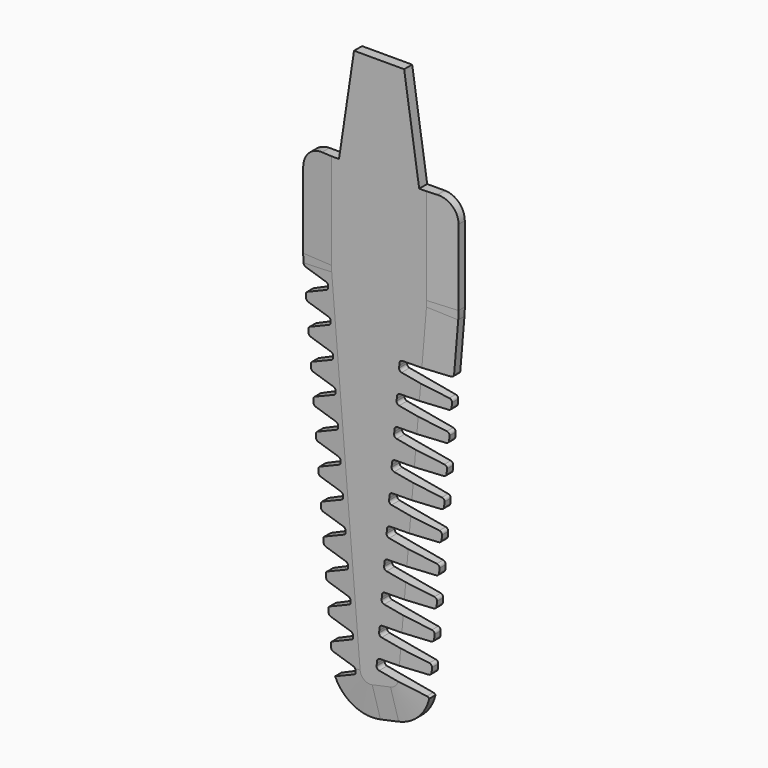
from build123d import *

# Parameters (mm, degrees)
F1_DEPTH    = 0.635
F2_T1_DEPTH = 3.9112557533
F3_R        = 2.54
F4_R        = 5.08
F11_DEPTH   = 12.7
F13_DEPTH   = 12.7
F15_DEPTH   = 12.7
F17_DEPTH   = 0.635
F20_DEPTH   = 12.7


# Not quite as in the source:
# - a fillet or chamfer that OpenCascade refuses, or shapes differently, is made with other operations: its cross-section is extruded or revolved along the edge and cut away or added
# - two fillets or chamfers of one size are made in one step


with BuildPart() as f1:
    # F0 (on Front) → F1 (new body, symmetric)
    with BuildSketch(Plane.XZ):
        Polygon((-9.8425, -12.7), (-5.715, -62.23), (5.9259355188, -59.6987737741), (9.8425, -12.7), (9.8425, 0), (3.175, 0), (0, 0), (-3.175, 0), (-9.8425, 0), align=None)
    extrude(amount=F1_DEPTH, both=True)

    # F2: fillet of radius 12.7 on 2 edges, made by hand

    # F2_s2 → F2_t1 (cut)
    with BuildSketch(Plane.XZ.offset(-1.9556278767)):
        with BuildLine():
            ThreePointArc((-9.7986311297, -13.2264264435), (-9.8315280429, -12.6995436261), (-9.8425, -12.1717488493))
            Line((-9.8425, -12.1717488493), (-9.8425, -12.7))
            Line((-9.8425, -12.7), (-9.7986311297, -13.2264264435))
        make_face()
        with BuildLine():
            ThreePointArc((9.8425, -12.1717488493), (9.8315280429, -12.6995436261), (9.7986311297, -13.2264264435))
            Line((9.7986311297, -13.2264264435), (9.8425, -12.7))
            Line((9.8425, -12.7), (9.8425, -12.1717488493))
        make_face()
    extrude(amount=F2_T1_DEPTH, mode=Mode.SUBTRACT)

    # F3
    f3_edges = [f1.edges().sort_by_distance(p)[0] for p in [
        (9.8425, 0, 0),
        (-9.8425, 0, 0),
    ]]
    fillet(f3_edges, radius=F3_R)

    # F4
    f4_edges = [f1.edges().sort_by_distance(p)[0] for p in [
        (-5.715, 0, -62.23),
        (5.925936, 0, -59.698774),
    ]]
    fillet(f4_edges, radius=F4_R)


with BuildPart() as f8:
    # F8: sweep along a path in F7
    with BuildLine(Plane.XZ) as f8_path:
        Line((9.8425, 0), (9.8425, -12.1717488493))
        ThreePointArc((9.8425, -12.1717488493), (9.8315280429, -12.6995436261), (9.7986311297, -13.2264264435))
        Line((9.7986311297, -13.2264264435), (6.2379260636, -55.9548872367))
        ThreePointArc((6.2379260636, -55.9548872367), (4.9949337053, -58.8823630896), (2.2548556559, -60.4970200672))
        Line((2.2548556559, -60.4970200672), (-0.0542502185, -60.9991162551))
        ThreePointArc((-0.0542502185, -60.9991162551), (-4.1542208032, -60.1195272618), (-6.1960847146, -56.4569834247))
        Line((-6.1960847146, -56.4569834247), (-9.7986311297, -13.2264264435))
        ThreePointArc((-9.7986311297, -13.2264264435), (-9.8315280429, -12.6995436261), (-9.8425, -12.1717488493))
        Line((-9.8425, -12.1717488493), (-9.8425, 1.6673188657))
    # F6 (on Top) → F8 (sweep)
    with BuildSketch(Plane.XY):
        Polygon((9.8425, -0.635), (9.8425, -0.34925), (6.0325, -0.635), align=None)
    sweep(path=f8_path.line)


with BuildPart() as f1_1:
    add(f1.part)

    # F9: cut F8
    add(f8.part, mode=Mode.SUBTRACT)

    # F10 (on Front) → F11 (cut, symmetric)
    with BuildSketch(Plane.XZ):
        Polygon((5.8208333333, -60.96), (-5.715, -62.23), (5.715, -62.23), align=None)
    extrude(amount=F11_DEPTH, both=True, mode=Mode.SUBTRACT)

    # F12 (on Front) → F13 (cut, symmetric)
    with BuildSketch(Plane.XZ):
        with BuildLine():
            ThreePointArc((5.8493657763, -56.4687369075), (6.0838454994, -56.6117604145), (6.1612256866, -56.8752917613))
            Line((6.1612256866, -56.8752917613), (6.4296508148, -53.6541902219))
            ThreePointArc((6.4296508148, -53.6541902219), (6.3097189591, -53.9012788985), (6.0548005827, -54.0035192306))
            Line((6.0548005827, -54.0035192306), (0.1109684718, -54.0789339927))
            ThreePointArc((0.1109684718, -54.0789339927), (-0.1439499045, -54.1811743248), (-0.2638817603, -54.4282630014))
            Line((-0.2638817603, -54.4282630014), (-0.2878708353, -54.7161319011))
            Line((-0.2878708353, -54.7161319011), (-0.3118599102, -55.0040008009))
            ThreePointArc((-0.3118599102, -55.0040008009), (-0.2344797231, -55.2675321477), (0, -55.4105556547))
            Line((0, -55.4105556547), (5.8493657763, -56.4687369075))
        make_face()
    extrude(amount=F13_DEPTH, both=True, mode=Mode.SUBTRACT)

    # F14 (on Front) → F15 (cut, symmetric)
    with BuildSketch(Plane.XZ):
        with BuildLine():
            ThreePointArc((6.4296508148, -53.6541902219), (6.3097189591, -53.9012788985), (6.0548005827, -54.0035192306))
            Line((6.0548005827, -54.0035192306), (0.1109684718, -54.0789339927))
            ThreePointArc((0.1109684718, -54.0789339927), (-0.1439499045, -54.1811743248), (-0.2638817603, -54.4282630014))
            Line((-0.2638817603, -54.4282630014), (-0.2878708353, -54.7161319011))
            Line((-0.2878708353, -54.7161319011), (-0.3118599102, -55.0040008009))
            ThreePointArc((-0.3118599102, -55.0040008009), (-0.2344797231, -55.2675321477), (0, -55.4105556547))
            Line((0, -55.4105556547), (5.8493657763, -56.4687369075))
            ThreePointArc((5.8493657763, -56.4687369075), (6.0838454994, -56.6117604145), (6.1612256866, -56.8752917613))
            Line((6.1612256866, -56.8752917613), (6.4296508148, -53.6541902219))
        make_face()
        with BuildLine():
            Line((6.4776289648, -53.0784524224), (6.7460540931, -49.857350883))
            ThreePointArc((6.7460540931, -49.857350883), (6.6261222373, -50.1044395596), (6.371203861, -50.2066798917))
            Line((6.371203861, -50.2066798917), (0.4273717501, -50.2820946538))
            ThreePointArc((0.4273717501, -50.2820946538), (0.1724533737, -50.3843349859), (0.052521518, -50.6314236625))
            Line((0.052521518, -50.6314236625), (0.028532443, -50.9192925622))
            Line((0.028532443, -50.9192925622), (0.004543368, -51.207161462))
            ThreePointArc((0.004543368, -51.207161462), (0.0819235551, -51.4706928088), (0.3164032782, -51.6137163158))
            Line((0.3164032782, -51.6137163158), (6.1657690546, -52.6718975686))
            ThreePointArc((6.1657690546, -52.6718975686), (6.4002487777, -52.8149210756), (6.4776289648, -53.0784524224))
        make_face()
        with BuildLine():
            Line((6.794032243, -49.2816130835), (7.0624573713, -46.0605115441))
            ThreePointArc((7.0624573713, -46.0605115441), (6.9425255156, -46.3076002207), (6.6876071392, -46.4098405527))
            Line((6.6876071392, -46.4098405527), (0.7437750283, -46.4852553149))
            ThreePointArc((0.7437750283, -46.4852553149), (0.4888566519, -46.587495647), (0.3689247962, -46.8345843236))
            Line((0.3689247962, -46.8345843236), (0.3449357212, -47.1224532233))
            Line((0.3449357212, -47.1224532233), (0.3209466463, -47.4103221231))
            ThreePointArc((0.3209466463, -47.4103221231), (0.3983268334, -47.6738534699), (0.6328065565, -47.8168769769))
            Line((0.6328065565, -47.8168769769), (6.4821723328, -48.8750582297))
            ThreePointArc((6.4821723328, -48.8750582297), (6.7166520559, -49.0180817367), (6.794032243, -49.2816130835))
        make_face()
        with BuildLine():
            Line((7.1104355213, -45.4847737446), (7.3788606496, -42.2636722052))
            ThreePointArc((7.3788606496, -42.2636722052), (7.2589287938, -42.5107608818), (7.0040104175, -42.6130012138))
            Line((7.0040104175, -42.6130012138), (1.0601783066, -42.688415976))
            ThreePointArc((1.0601783066, -42.688415976), (0.8052599302, -42.7906563081), (0.6853280745, -43.0377449846))
            Line((0.6853280745, -43.0377449846), (0.6613389995, -43.3256138844))
            Line((0.6613389995, -43.3256138844), (0.6373499245, -43.6134827841))
            ThreePointArc((0.6373499245, -43.6134827841), (0.7147301116, -43.877014131), (0.9492098347, -44.020037638))
            Line((0.9492098347, -44.020037638), (6.7985756111, -45.0782188908))
            ThreePointArc((6.7985756111, -45.0782188908), (7.0330553342, -45.2212423978), (7.1104355213, -45.4847737446))
        make_face()
        with BuildLine():
            Line((7.4268387995, -41.6879344057), (7.6952639278, -38.4668328663))
            ThreePointArc((7.6952639278, -38.4668328663), (7.5753320721, -38.7139215429), (7.3204136957, -38.8161618749))
            Line((7.3204136957, -38.8161618749), (1.3765815848, -38.8915766371))
            ThreePointArc((1.3765815848, -38.8915766371), (1.1216632084, -38.9938169692), (1.0017313527, -39.2409056457))
            Line((1.0017313527, -39.2409056457), (0.9777422777, -39.5287745455))
            Line((0.9777422777, -39.5287745455), (0.9537532027, -39.8166434452))
            ThreePointArc((0.9537532027, -39.8166434452), (1.0311333899, -40.080174792), (1.265613113, -40.2231982991))
            Line((1.265613113, -40.2231982991), (7.1149788893, -41.2813795518))
            ThreePointArc((7.1149788893, -41.2813795518), (7.3494586124, -41.4244030589), (7.4268387995, -41.6879344057))
        make_face()
        with BuildLine():
            Line((7.7432420778, -37.8910950668), (8.0116672061, -34.6699935274))
            ThreePointArc((8.0116672061, -34.6699935274), (7.8917353503, -34.9170822039), (7.636816974, -35.019322536))
            Line((7.636816974, -35.019322536), (1.692984863, -35.0947372982))
            ThreePointArc((1.692984863, -35.0947372982), (1.4380664867, -35.1969776302), (1.3181346309, -35.4440663068))
            Line((1.3181346309, -35.4440663068), (1.294145556, -35.7319352066))
            Line((1.294145556, -35.7319352066), (1.270156481, -36.0198041063))
            ThreePointArc((1.270156481, -36.0198041063), (1.3475366681, -36.2833354531), (1.5820163912, -36.4263589602))
            Line((1.5820163912, -36.4263589602), (7.4313821675, -37.4845402129))
            ThreePointArc((7.4313821675, -37.4845402129), (7.6658618907, -37.62756372), (7.7432420778, -37.8910950668))
        make_face()
        with BuildLine():
            Line((8.059645356, -34.0942557279), (8.3280704843, -30.8731541885))
            ThreePointArc((8.3280704843, -30.8731541885), (8.2081386286, -31.120242865), (7.9532202522, -31.2224831971))
            Line((7.9532202522, -31.2224831971), (2.0093881413, -31.2978979593))
            ThreePointArc((2.0093881413, -31.2978979593), (1.7544697649, -31.4001382913), (1.6345379092, -31.6472269679))
            Line((1.6345379092, -31.6472269679), (1.6105488342, -31.9350958677))
            Line((1.6105488342, -31.9350958677), (1.5865597592, -32.2229647674))
            ThreePointArc((1.5865597592, -32.2229647674), (1.6639399463, -32.4864961142), (1.8984196695, -32.6295196212))
            Line((1.8984196695, -32.6295196212), (7.7477854458, -33.687700874))
            ThreePointArc((7.7477854458, -33.687700874), (7.9822651689, -33.830724381), (8.059645356, -34.0942557279))
        make_face()
        with BuildLine():
            Line((8.3760486343, -30.2974163889), (8.6444737625, -27.0763148495))
            ThreePointArc((8.6444737625, -27.0763148495), (8.5245419068, -27.3234035261), (8.2696235304, -27.4256438582))
            Line((8.2696235304, -27.4256438582), (2.3257914195, -27.5010586203))
            ThreePointArc((2.3257914195, -27.5010586203), (2.0708730432, -27.6032989524), (1.9509411874, -27.850387629))
            Line((1.9509411874, -27.850387629), (1.9269521124, -28.1382565287))
            Line((1.9269521124, -28.1382565287), (1.9029630375, -28.4261254285))
            ThreePointArc((1.9029630375, -28.4261254285), (1.9803432246, -28.6896567753), (2.2148229477, -28.8326802823))
            Line((2.2148229477, -28.8326802823), (8.064188724, -29.8908615351))
            ThreePointArc((8.064188724, -29.8908615351), (8.2986684471, -30.0338850421), (8.3760486343, -30.2974163889))
        make_face()
        with BuildLine():
            Line((8.6924519125, -26.50057705), (8.9608770408, -23.2794755106))
            ThreePointArc((8.9608770408, -23.2794755106), (8.840945185, -23.5265641872), (8.5860268087, -23.6288045193))
            Line((8.5860268087, -23.6288045193), (2.6421946978, -23.7042192814))
            ThreePointArc((2.6421946978, -23.7042192814), (2.3872763214, -23.8064596135), (2.2673444657, -24.0535482901))
            Line((2.2673444657, -24.0535482901), (2.2433553907, -24.3414171898))
            Line((2.2433553907, -24.3414171898), (2.2193663157, -24.6292860896))
            ThreePointArc((2.2193663157, -24.6292860896), (2.2967465028, -24.8928174364), (2.5312262259, -25.0358409434))
            Line((2.5312262259, -25.0358409434), (8.3805920023, -26.0940221962))
            ThreePointArc((8.3805920023, -26.0940221962), (8.6150717254, -26.2370457032), (8.6924519125, -26.50057705))
        make_face()
        with BuildLine():
            Line((9.0088551907, -22.7037377111), (9.277280319, -19.4826361717))
            ThreePointArc((9.277280319, -19.4826361717), (9.1573484633, -19.7297248483), (8.9024300869, -19.8319651804))
            Line((8.9024300869, -19.8319651804), (2.958597976, -19.9073799425))
            ThreePointArc((2.958597976, -19.9073799425), (2.7036795996, -20.0096202746), (2.5837477439, -20.2567089512))
            Line((2.5837477439, -20.2567089512), (2.5597586689, -20.5445778509))
            Line((2.5597586689, -20.5445778509), (2.535769594, -20.8324467507))
            ThreePointArc((2.535769594, -20.8324467507), (2.6131497811, -21.0959780975), (2.8476295042, -21.2390016045))
            Line((2.8476295042, -21.2390016045), (8.6969952805, -22.2971828573))
            ThreePointArc((8.6969952805, -22.2971828573), (8.9314750036, -22.4402063643), (9.0088551907, -22.7037377111))
        make_face()
    extrude(amount=F15_DEPTH, both=True, mode=Mode.SUBTRACT)

    # F16 (on Front) → F17 (join, symmetric)
    with BuildSketch(Plane.XZ):
        Polygon((-3.175, 12.7), (-5.08, 0), (0, 0), (5.08, 0), (3.175, 12.7), align=None)
    extrude(amount=F17_DEPTH, both=True)

    # F19 (on Front) → F20 (cut, symmetric)
    with BuildSketch(Plane.XZ):
        with BuildLine():
            Line((-6.3161662287, -55.0160052561), (-6.0314032782, -58.4331606611))
            ThreePointArc((-6.0314032782, -58.4331606611), (-5.9789942026, -58.2064506864), (-5.8045136998, -58.0525004413))
            Line((-5.8045136998, -58.0525004413), (-3.2296659927, -56.925280461))
            ThreePointArc((-3.2296659927, -56.925280461), (-3.0551854899, -56.771330216), (-3.0027764143, -56.5446202413))
            Line((-3.0027764143, -56.5446202413), (-3.0167275278, -56.3772068788))
            ThreePointArc((-3.0167275278, -56.3772068788), (-3.1059381292, -56.1622985438), (-3.3034934243, -56.039351282))
            Line((-3.3034934243, -56.039351282), (-6.0294003321, -55.3538608529))
            ThreePointArc((-6.0294003321, -55.3538608529), (-6.2269556273, -55.230913591), (-6.3161662287, -55.0160052561))
        make_face()
        with BuildLine():
            Line((-6.6325695069, -51.2191659172), (-6.3478065565, -54.6363213222))
            ThreePointArc((-6.3478065565, -54.6363213222), (-6.2953974809, -54.4096113475), (-6.120916978, -54.2556611024))
            Line((-6.120916978, -54.2556611024), (-3.546069271, -53.1284411221))
            ThreePointArc((-3.546069271, -53.1284411221), (-3.3715887681, -52.9744908771), (-3.3191796925, -52.7477809024))
            Line((-3.3191796925, -52.7477809024), (-3.333130806, -52.5803675399))
            ThreePointArc((-3.333130806, -52.5803675399), (-3.4223414074, -52.3654592049), (-3.6198967026, -52.242511943))
            Line((-3.6198967026, -52.242511943), (-6.3458036104, -51.557021514))
            ThreePointArc((-6.3458036104, -51.557021514), (-6.5433589055, -51.4340742521), (-6.6325695069, -51.2191659172))
        make_face()
        with BuildLine():
            Line((-6.9489727851, -47.4223265782), (-6.6642098347, -50.8394819833))
            ThreePointArc((-6.6642098347, -50.8394819833), (-6.6118007591, -50.6127720086), (-6.4373202563, -50.4588217635))
            Line((-6.4373202563, -50.4588217635), (-3.8624725492, -49.3316017832))
            ThreePointArc((-3.8624725492, -49.3316017832), (-3.6879920463, -49.1776515382), (-3.6355829707, -48.9509415635))
            Line((-3.6355829707, -48.9509415635), (-3.6495340843, -48.783528201))
            ThreePointArc((-3.6495340843, -48.783528201), (-3.7387446857, -48.568619866), (-3.9362999808, -48.4456726041))
            Line((-3.9362999808, -48.4456726041), (-6.6622068886, -47.7601821751))
            ThreePointArc((-6.6622068886, -47.7601821751), (-6.8597621837, -47.6372349132), (-6.9489727851, -47.4223265782))
        make_face()
        with BuildLine():
            Line((-7.2653760634, -43.6254872393), (-6.980613113, -47.0426426443))
            ThreePointArc((-6.980613113, -47.0426426443), (-6.9282040374, -46.8159326697), (-6.7537235345, -46.6619824246))
            Line((-6.7537235345, -46.6619824246), (-4.1788758275, -45.5347624443))
            ThreePointArc((-4.1788758275, -45.5347624443), (-4.0043953246, -45.3808121993), (-3.951986249, -45.1541022246))
            Line((-3.951986249, -45.1541022246), (-3.9659373625, -44.986688862))
            ThreePointArc((-3.9659373625, -44.986688862), (-4.0551479639, -44.7717805271), (-4.252703259, -44.6488332652))
            Line((-4.252703259, -44.6488332652), (-6.9786101669, -43.9633428361))
            ThreePointArc((-6.9786101669, -43.9633428361), (-7.176165462, -43.8403955743), (-7.2653760634, -43.6254872393))
        make_face()
        with BuildLine():
            Line((-7.5817793416, -39.8286479004), (-7.2970163912, -43.2458033054))
            ThreePointArc((-7.2970163912, -43.2458033054), (-7.2446073156, -43.0190933307), (-7.0701268127, -42.8651430857))
            Line((-7.0701268127, -42.8651430857), (-4.4952791057, -41.7379231054))
            ThreePointArc((-4.4952791057, -41.7379231054), (-4.3207986028, -41.5839728603), (-4.2683895272, -41.3572628856))
            Line((-4.2683895272, -41.3572628856), (-4.2823406408, -41.1898495231))
            ThreePointArc((-4.2823406408, -41.1898495231), (-4.3715512422, -40.9749411882), (-4.5691065373, -40.8519939263))
            Line((-4.5691065373, -40.8519939263), (-7.2950134451, -40.1665034972))
            ThreePointArc((-7.2950134451, -40.1665034972), (-7.4925687402, -40.0435562354), (-7.5817793416, -39.8286479004))
        make_face()
        with BuildLine():
            Line((-7.8981826199, -36.0318085615), (-7.6134196695, -39.4489639665))
            ThreePointArc((-7.6134196695, -39.4489639665), (-7.5610105939, -39.2222539918), (-7.386530091, -39.0683037468))
            Line((-7.386530091, -39.0683037468), (-4.8116823839, -37.9410837665))
            ThreePointArc((-4.8116823839, -37.9410837665), (-4.6372018811, -37.7871335214), (-4.5847928055, -37.5604235467))
            Line((-4.5847928055, -37.5604235467), (-4.598743919, -37.3930101842))
            ThreePointArc((-4.598743919, -37.3930101842), (-4.6879545204, -37.1781018493), (-4.8855098155, -37.0551545874))
            Line((-4.8855098155, -37.0551545874), (-7.6114167234, -36.3696641583))
            ThreePointArc((-7.6114167234, -36.3696641583), (-7.8089720185, -36.2467168964), (-7.8981826199, -36.0318085615))
        make_face()
        with BuildLine():
            Line((-8.2145858981, -32.2349692226), (-7.9298229477, -35.6521246276))
            ThreePointArc((-7.9298229477, -35.6521246276), (-7.8774138721, -35.4254146529), (-7.7029333692, -35.2714644079))
            Line((-7.7029333692, -35.2714644079), (-5.1280856622, -34.1442444276))
            ThreePointArc((-5.1280856622, -34.1442444276), (-4.9536051593, -33.9902941825), (-4.9011960837, -33.7635842078))
            Line((-4.9011960837, -33.7635842078), (-4.9151471973, -33.5961708453))
            ThreePointArc((-4.9151471973, -33.5961708453), (-5.0043577987, -33.3812625104), (-5.2019130938, -33.2583152485))
            Line((-5.2019130938, -33.2583152485), (-7.9278200016, -32.5728248194))
            ThreePointArc((-7.9278200016, -32.5728248194), (-8.1253752967, -32.4498775575), (-8.2145858981, -32.2349692226))
        make_face()
        with BuildLine():
            Line((-8.5309891764, -28.4381298837), (-8.2462262259, -31.8552852887))
            ThreePointArc((-8.2462262259, -31.8552852887), (-8.1938171503, -31.628575314), (-8.0193366475, -31.474625069))
            Line((-8.0193366475, -31.474625069), (-5.4444889404, -30.3474050886))
            ThreePointArc((-5.4444889404, -30.3474050886), (-5.2700084376, -30.1934548436), (-5.217599362, -29.9667448689))
            Line((-5.217599362, -29.9667448689), (-5.2315504755, -29.7993315064))
            ThreePointArc((-5.2315504755, -29.7993315064), (-5.3207610769, -29.5844231714), (-5.518316372, -29.4614759096))
            Line((-5.518316372, -29.4614759096), (-8.2442232798, -28.7759854805))
            ThreePointArc((-8.2442232798, -28.7759854805), (-8.441778575, -28.6530382186), (-8.5309891764, -28.4381298837))
        make_face()
        with BuildLine():
            Line((-8.8473924546, -24.6412905448), (-8.5626295042, -28.0584459498))
            ThreePointArc((-8.5626295042, -28.0584459498), (-8.5102204286, -27.8317359751), (-8.3357399257, -27.67778573))
            Line((-8.3357399257, -27.67778573), (-5.7608922187, -26.5505657497))
            ThreePointArc((-5.7608922187, -26.5505657497), (-5.5864117158, -26.3966155047), (-5.5340026402, -26.16990553))
            Line((-5.5340026402, -26.16990553), (-5.5479537537, -26.0024921675))
            ThreePointArc((-5.5479537537, -26.0024921675), (-5.6371643551, -25.7875838325), (-5.8347196503, -25.6646365707))
            Line((-5.8347196503, -25.6646365707), (-8.5606265581, -24.9791461416))
            ThreePointArc((-8.5606265581, -24.9791461416), (-8.7581818532, -24.8561988797), (-8.8473924546, -24.6412905448))
        make_face()
        with BuildLine():
            Line((-9.1637957328, -20.8444512058), (-8.8790327824, -24.2616066109))
            ThreePointArc((-8.8790327824, -24.2616066109), (-8.8266237068, -24.0348966362), (-8.652143204, -23.8809463911))
            Line((-8.652143204, -23.8809463911), (-6.0772954969, -22.7537264108))
            ThreePointArc((-6.0772954969, -22.7537264108), (-5.902814994, -22.5997761658), (-5.8504059184, -22.3730661911))
            Line((-5.8504059184, -22.3730661911), (-5.864357032, -22.2056528286))
            ThreePointArc((-5.864357032, -22.2056528286), (-5.9535676334, -21.9907444936), (-6.1511229285, -21.8677972317))
            Line((-6.1511229285, -21.8677972317), (-8.8770298363, -21.1823068027))
            ThreePointArc((-8.8770298363, -21.1823068027), (-9.0745851314, -21.0593595408), (-9.1637957328, -20.8444512058))
        make_face()
        with BuildLine():
            Line((-9.4801990111, -17.0476118669), (-9.1954360607, -20.464767272))
            ThreePointArc((-9.1954360607, -20.464767272), (-9.1430269851, -20.2380572973), (-8.9685464822, -20.0841070522))
            Line((-8.9685464822, -20.0841070522), (-6.3936987752, -18.9568870719))
            ThreePointArc((-6.3936987752, -18.9568870719), (-6.2192182723, -18.8029368269), (-6.1668091967, -18.5762268522))
            Line((-6.1668091967, -18.5762268522), (-6.1807603102, -18.4088134897))
            ThreePointArc((-6.1807603102, -18.4088134897), (-6.2699709116, -18.1939051547), (-6.4675262067, -18.0709578928))
            Line((-6.4675262067, -18.0709578928), (-9.1934331146, -17.3854674638))
            ThreePointArc((-9.1934331146, -17.3854674638), (-9.3909884097, -17.2625202019), (-9.4801990111, -17.0476118669))
        make_face()
        with BuildLine():
            Line((-9.7966022893, -13.250772528), (-9.5118393389, -16.667927933))
            ThreePointArc((-9.5118393389, -16.667927933), (-9.4594302633, -16.4412179583), (-9.2849497604, -16.2872677133))
            Line((-9.2849497604, -16.2872677133), (-6.7101020534, -15.160047733))
            ThreePointArc((-6.7101020534, -15.160047733), (-6.5356215505, -15.006097488), (-6.4832124749, -14.7793875133))
            Line((-6.4832124749, -14.7793875133), (-6.4971635885, -14.6119741507))
            ThreePointArc((-6.4971635885, -14.6119741507), (-6.5863741899, -14.3970658158), (-6.783929485, -14.2741185539))
            Line((-6.783929485, -14.2741185539), (-9.5098363928, -13.5886281248))
            ThreePointArc((-9.5098363928, -13.5886281248), (-9.7073916879, -13.465680863), (-9.7966022893, -13.250772528))
        make_face()
    extrude(amount=F20_DEPTH, both=True, mode=Mode.SUBTRACT)


solid = f1_1.part
